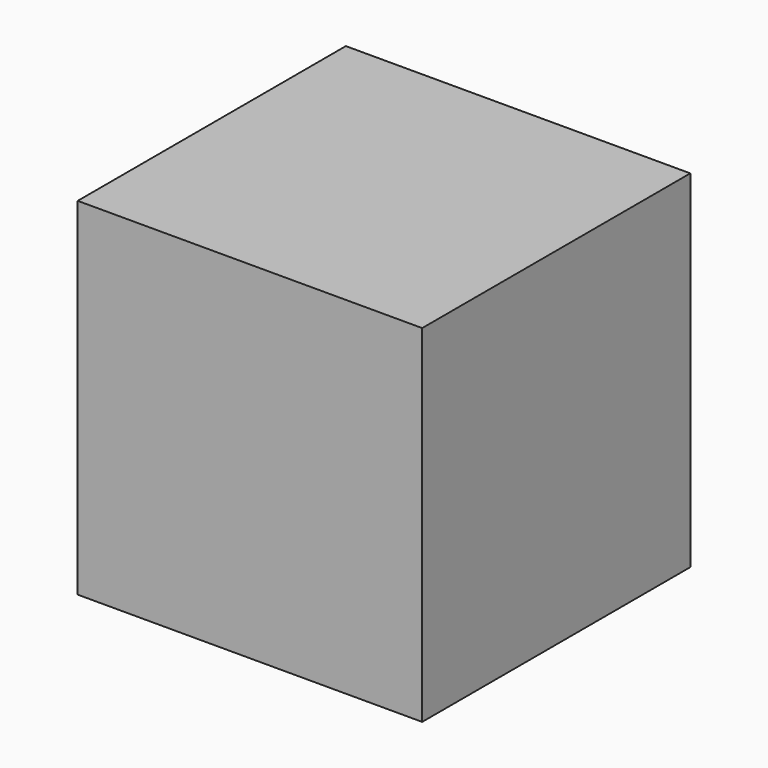
from build123d import *

# Parameters (mm, degrees)
F0_W         = 156.6458195448
F0_H         = 157.6596796513
F1_DEPTH     = 76.2
F3_DEPTH     = 5.334
F2_W         = 43.3532558382
F2_H         = 43.0700061843
F4_TEXT_SIZE = 8.609793925
F5_DEPTH     = 1.27


# Not quite as in the source:
# - Text() gives the source's letters only with a copy of the font that has no kerning and outlines rounded to 1/6400 em; it was checked with that copy


with BuildPart() as f1:
    # F0 (on Front) → F1 (new body, symmetric)
    with BuildSketch(Plane.XZ):
        with Locations((-2.6825293899, -3.1860098243)):
            Rectangle(F0_W, F0_H)
    extrude(amount=F1_DEPTH, both=True)

    # F4 (on face) → F5 (join)
    with BuildSketch(Plane(origin=(0, 0, -82.0158496499), x_dir=(1, 0, 0), z_dir=(0, 0, -1))):
        with Locations((-50.5685638636, 0)):
            Text('Made By: Daniel Tolner', F4_TEXT_SIZE, font='Open Sans', text_align=(TextAlign.LEFT, TextAlign.BOTTOM))
    extrude(amount=F5_DEPTH)


with BuildPart() as f3:
    # F2 (on face) → F3 (new body)
    with BuildSketch(Plane(origin=(-81.0054391623, 0, 0), x_dir=(0, -1, 0), z_dir=(-1, 0, 0))):
        Polygon((19.3002615124, 8.0148773268), (-19.9526809156, 8.0148773268), (-19.9526809156, -9.0763079934), (-19.9526809156, -26.1674933136), (19.3002615124, -26.1674933136), align=None)
        Polygon((-19.9526809156, -26.1674933136), (-19.9526809156, -9.0763079934), (-45.2771559358, -9.0763079934), (-45.2771559358, -69.546058774), (-19.9526809156, -69.546058774), align=None)
    extrude(amount=F3_DEPTH)


with BuildPart() as f3b:
    # F2 (on face) → F3, piece 2 (new body)
    with BuildSketch(Plane(origin=(-81.0054391623, 0, 0), x_dir=(0, -1, 0), z_dir=(-1, 0, 0))):
        with Locations((-41.6293088347, 29.5498804189)):
            Rectangle(F2_W, F2_H)
    extrude(amount=F3_DEPTH)


with BuildPart() as f3c:
    # F2 (on face) → F3, piece 3 (new body)
    with BuildSketch(Plane(origin=(-81.0054391623, 0, 0), x_dir=(0, -1, 0), z_dir=(-1, 0, 0))):
        with Locations((41.6293088347, 29.5498804189)):
            Rectangle(F2_W, F2_H)
    extrude(amount=F3_DEPTH)


with BuildPart() as f3d:
    # F2 (on face) → F3, piece 4 (new body)
    with BuildSketch(Plane(origin=(-81.0054391623, 0, 0), x_dir=(0, -1, 0), z_dir=(-1, 0, 0))):
        Polygon((45.2771559358, -9.0763079934), (19.9526809156, -9.0763079934), (19.9526809156, -26.1674933136), (19.9526809156, -69.546058774), (45.2771559358, -69.546058774), align=None)
    extrude(amount=F3_DEPTH)


solid = Compound([f1.part, f3.part, f3b.part, f3c.part, f3d.part])
